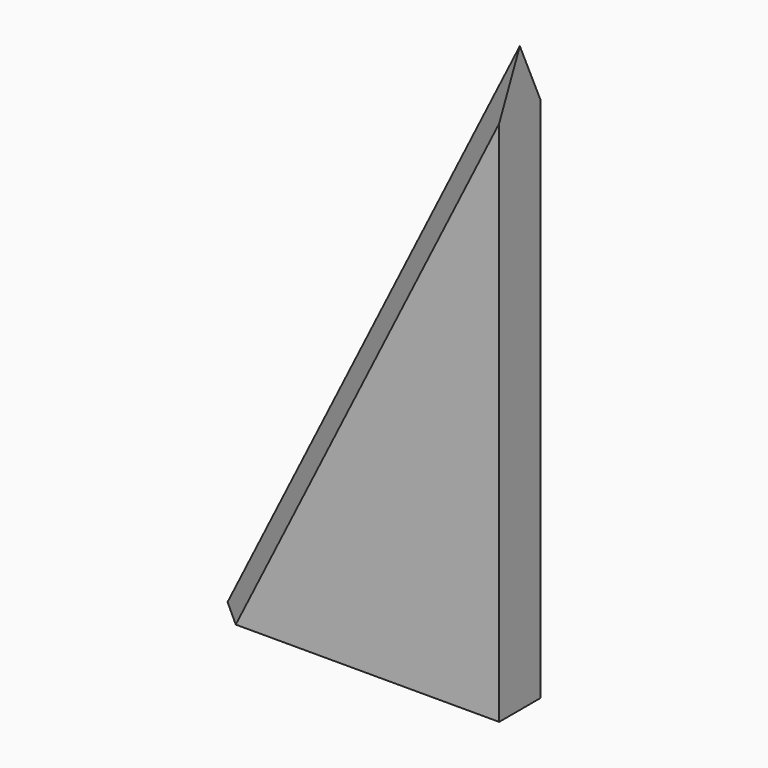
from build123d import *

# Parameters (mm, degrees)
F1_DEPTH    = 6.35
F2_T1_DEPTH = 111.3224891005


# Not quite as in the source:
# - a fillet or chamfer that OpenCascade refuses, or shapes differently, is made with other operations: its cross-section is extruded or revolved along the edge and cut away or added


with BuildPart() as f1:
    # F0 (on Front) → F1 (new body)
    with BuildSketch(Plane.XZ):
        Polygon((38.1, 76.2), (0, 0), (38.1, 0), align=None)
    extrude(amount=F1_DEPTH)

    # F2: chamfer of 5.08 on 2 edges, made by hand

    # F2_s2 → F2_t1 (cut)
    with BuildSketch(Plane(origin=(43.9424653053, 0, 87.8849306106), x_dir=(0, 1, 0), z_dir=(-0.4472135955, 0, -0.894427191))):
        Polygon((-1.27, 0), (-6.35, 5.08), (-6.35, 0), align=None)
        Polygon((-5.08, 0), (0, 5.08), (0, 0), align=None)
    extrude(amount=F2_T1_DEPTH, mode=Mode.SUBTRACT)


solid = f1.part
